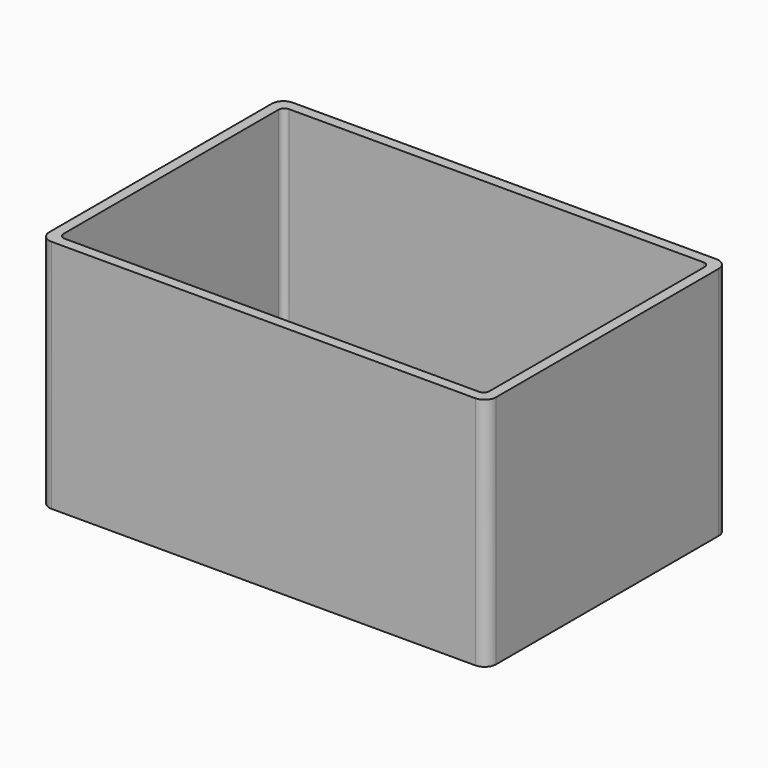
from build123d import *

# Parameters (mm, degrees)
F1_DEPTH = 40.64
F3_DEPTH = 38.608


# Not quite as in the source:
# - a feature names something its author has since deleted; it is built from what else it names


with BuildPart() as f1:
    # F0 (on Top) → F1 (new body)
    with BuildSketch(Plane.XY):
        with BuildLine():
            ThreePointArc((0, 2), (0.5857864376, 0.5857864376), (2, 0))
            Line((2, 0), (75.216, 0))
            ThreePointArc((75.216, 0), (76.6302135624, 0.5857864376), (77.216, 2))
            Line((77.216, 2), (77.216, 50.07))
            ThreePointArc((77.216, 50.07), (76.6302135624, 51.4842135624), (75.216, 52.07))
            Line((75.216, 52.07), (2, 52.07))
            ThreePointArc((2, 52.07), (0.5857864376, 51.4842135624), (0, 50.07))
            Line((0, 50.07), (0, 2))
        make_face()
    extrude(amount=F1_DEPTH)

    # F2 (on face) → F3 (cut)
    with BuildSketch(Plane.XY.offset(40.64)):
        with BuildLine():
            Line((74.416, 50.27), (2.8, 50.27))
            ThreePointArc((2.8, 50.27), (2.0928932188, 49.9771067812), (1.8, 49.27))
            Line((1.8, 49.27), (1.8, 2.8))
            ThreePointArc((1.8, 2.8), (2.0928932188, 2.0928932188), (2.8, 1.8))
            Line((2.8, 1.8), (74.416, 1.8))
            ThreePointArc((74.416, 1.8), (75.1231067812, 2.0928932188), (75.416, 2.8))
            Line((75.416, 2.8), (75.416, 49.27))
            ThreePointArc((75.416, 49.27), (75.1231067812, 49.9771067812), (74.416, 50.27))
        make_face()
    extrude(amount=-F3_DEPTH, mode=Mode.SUBTRACT)


solid = f1.part
